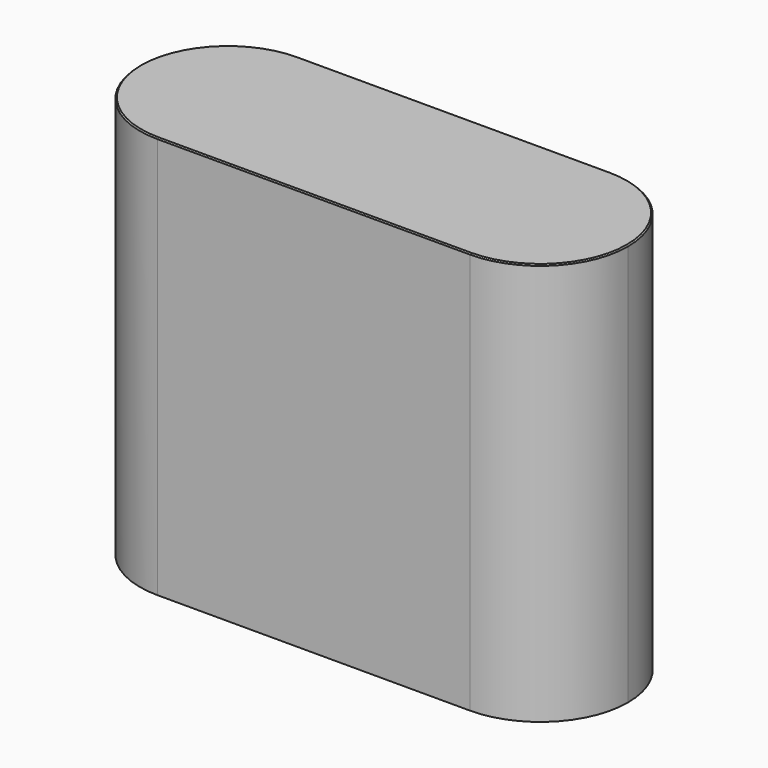
from build123d import *

# Parameters (mm, degrees)
F4_T     = -1.2
F5_SIZE  = 0.5
F6_W     = 3.6
F6_H     = 11.6
F7_DEPTH = 5


with BuildPart() as f3:
    # F2 (on offset) → F3 section 0
    with BuildSketch(Plane.XY.offset(165)):
        with BuildLine():
            Line((-64, -36), (64, -36))
            ThreePointArc((64, -36), (89.4558441227, -25.4558441227), (100, 0))
            ThreePointArc((100, 0), (89.4558441227, 25.4558441227), (64, 36))
            Line((64, 36), (-64, 36))
            ThreePointArc((-64, 36), (-89.4558441227, 25.4558441227), (-100, 0))
            ThreePointArc((-100, 0), (-89.4558441227, -25.4558441227), (-64, -36))
        make_face()
    # F0 (on Top) → F3 section 1
    with BuildSketch(Plane.XY):
        with BuildLine():
            Line((-64, -36), (64, -36))
            ThreePointArc((64, -36), (89.4558441227, -25.4558441227), (100, 0))
            ThreePointArc((100, 0), (89.4558441227, 25.4558441227), (64, 36))
            Line((64, 36), (-64, 36))
            ThreePointArc((-64, 36), (-89.4558441227, 25.4558441227), (-100, 0))
            ThreePointArc((-100, 0), (-89.4558441227, -25.4558441227), (-64, -36))
        make_face()
    loft()

    # F4
    f4_openings = [f3.faces().sort_by_distance(p)[0] for p in [
        (0, 0, 0),
    ]]
    offset(amount=F4_T, openings=f4_openings)

    # F5
    f5_edges = [f3.edges().sort_by_distance(p)[0] for p in [
        (-100, 0, 165),
        (0, 36, 165),
        (100, 0, 165),
        (0, -36, 165),
        (-98.8, 0, 163.8),
        (0, -34.8, 163.8),
        (98.8, 0, 163.8),
        (0, 34.8, 163.8),
    ]]
    chamfer(f5_edges, length=F5_SIZE)

    # F6 (on face) → F7 (join)
    with BuildSketch(Plane(origin=(0, 0, 163.8), x_dir=(1, 0, 0), z_dir=(0, 0, -1))):
        Rectangle(F6_W, F6_H)
    extrude(amount=F7_DEPTH)


solid = f3.part
